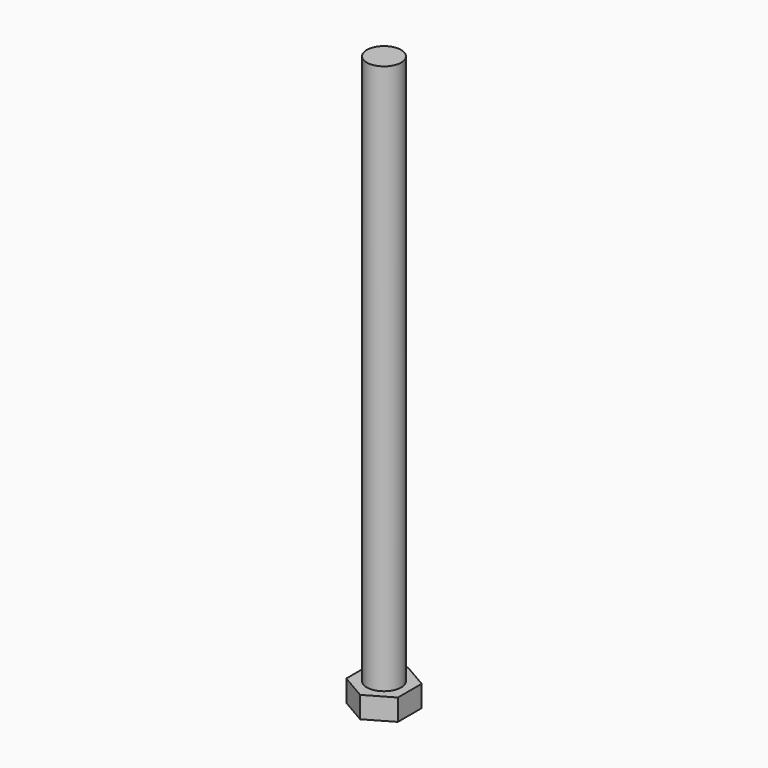
from build123d import *

# Parameters (mm, degrees)
F1_R     = 6.35
F2_DEPTH = 7.9375
F3_DEPTH = 211.1375


# Not quite as in the source:
# - a variable given as a bare number and used for a length is read in inches; the dataset says mm whatever the document's units were


with BuildPart() as f2:
    # F1 (on Top) → F2 (new body)
    with BuildSketch(Plane.XY):
        Polygon((9.525, -5.499261314), (9.525, 5.499261314), (0, 10.9985226281), (-9.525, 5.499261314), (-9.525, -5.499261314), (0, -10.9985226281), align=None)
        Circle(F1_R, mode=Mode.SUBTRACT)
    extrude(amount=F2_DEPTH)

    # F1 (on Top) → F3 (join)
    with BuildSketch(Plane.XY):
        Circle(F1_R)
    extrude(amount=F3_DEPTH)


solid = f2.part
